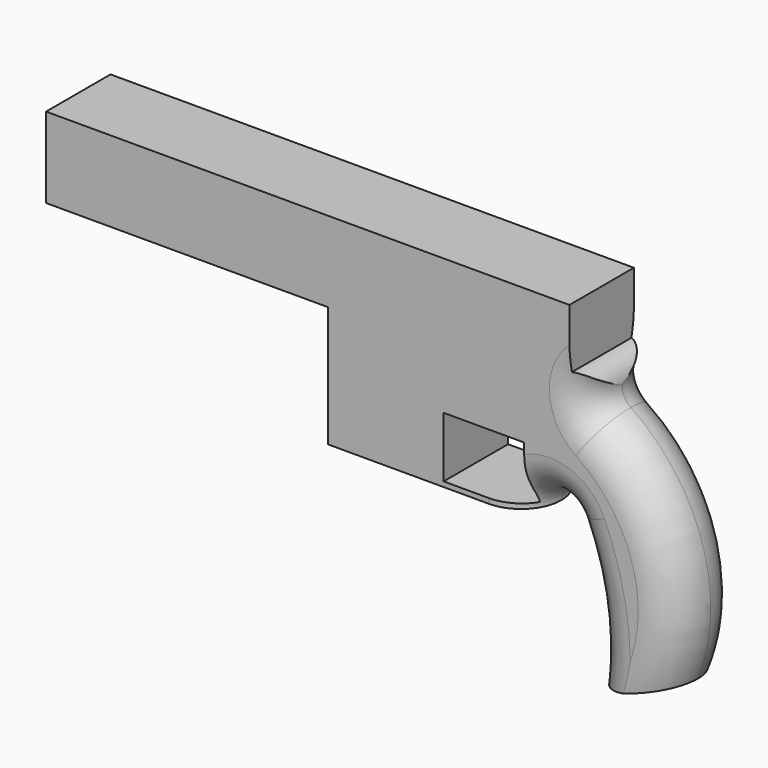
from build123d import *

# Parameters (mm, degrees)
F0_W         = 50.8
F0_H         = 38.1
F1_DEPTH     = 50.8
F2_T2_ANGLE  = 53.6002837339
F2_T4_ANGLE  = 53.6002837339
F2_T6_ANGLE  = 109.3939294159
F2_T8_ANGLE  = 109.3939294159
F2_T10_ANGLE = 342.5650608066
F2_T12_ANGLE = 342.5650608066
F2_T14_ANGLE = 359.64
F2_T16_ANGLE = 359.64


# Not quite as in the source:
# - a fillet or chamfer that OpenCascade refuses, or shapes differently, is made with other operations: its cross-section is extruded or revolved along the edge and cut away or added


with BuildPart() as f1:
    # F0 (on Front) → F1 (new body)
    with BuildSketch(Plane.XZ):
        with BuildLine():
            Line((-177.8, 0), (0, 0))
            Line((0, 0), (0, -76.2))
            Line((0, -76.2), (127, -76.2))
            ThreePointArc((127, -76.2), (137.069140052, -63.7754848813), (151.3100119581, -71.0524158741))
            ThreePointArc((151.3100119581, -71.0524158741), (163.8205179064, -114.6223435958), (164.0100119581, -159.9524158741))
            Line((164.0100119581, -159.9524158741), (213.1969004549, -147.2524158741))
            ThreePointArc((213.1969004549, -147.2524158741), (216.0088779453, -71.4162966266), (170.7058872965, -10.53392448))
            ThreePointArc((170.7058872965, -10.53392448), (166.5887281869, -5.9663543586), (165.1, 0))
            ThreePointArc((165.1, 0), (161.3802561211, 8.9802561211), (152.4, 12.7))
            Line((152.4, 12.7), (152.4, 50.8))
            Line((152.4, 50.8), (-177.8, 50.8))
            Line((-177.8, 50.8), (-177.8, 0))
        make_face()
        with Locations((98.425, -53.975)):
            Rectangle(F0_W, F0_H, mode=Mode.SUBTRACT)
    extrude(amount=F1_DEPTH)

    # F2: fillet of radius 25.4 on 8 edges, made by hand

    # F2_s1 → F2_t2 (revolve, cut)
    with BuildSketch(Plane(origin=(51.1854271814, 0, -115.4451111674), x_dir=(0, 1, 0), z_dir=(-0.4053215847, 0, 0.9141741699))):
        with BuildLine():
            ThreePointArc((-25.4, -109.5246267837), (-43.3605122421, -116.9641145416), (-50.8, -134.9246267837))
            Line((-50.8, -134.9246267837), (-50.8, -109.5246267837))
            Line((-50.8, -109.5246267837), (-25.4, -109.5246267837))
        make_face()
    revolve(axis=Axis((0.3798565029, -50.8, -137.9710095106), (0, 1, 0)), revolution_arc=F2_T2_ANGLE, mode=Mode.SUBTRACT)

    # F2_s3 → F2_t4 (revolve, cut)
    with BuildSketch(Plane(origin=(51.1854271814, 0, -115.4451111674), x_dir=(0, 1, 0), z_dir=(-0.4053215847, 0, 0.9141741699))):
        with BuildLine():
            ThreePointArc((-25.4, -109.5246267837), (-7.4394877579, -116.9641145416), (0, -134.9246267837))
            Line((0, -134.9246267837), (0, -109.5246267837))
            Line((0, -109.5246267837), (-25.4, -109.5246267837))
        make_face()
    revolve(axis=Axis((0.3798565029, 0, -137.9710095106), (0, 1, 0)), revolution_arc=F2_T4_ANGLE, mode=Mode.SUBTRACT)

    # F2_s5 → F2_t6 (revolve, cut)
    with BuildSketch(Plane(origin=(18.3403057366, 0, 13.6443784603), x_dir=(0, 1, 0), z_dir=(-0.802321654, 0, -0.5968919194))):
        with BuildLine():
            ThreePointArc((-25.4, 262.599154914), (-43.3605122421, 255.1596671561), (-50.8, 237.199154914))
            Line((-50.8, 237.199154914), (-50.8, 262.599154914))
            Line((-50.8, 262.599154914), (-25.4, 262.599154914))
        make_face()
    revolve(axis=Axis((106.8588729648, -50.8, -105.3392447997), (0, -1, 0)), revolution_arc=F2_T6_ANGLE, mode=Mode.SUBTRACT)

    # F2_s7 → F2_t8 (revolve, cut)
    with BuildSketch(Plane(origin=(18.3403057366, 0, 13.6443784603), x_dir=(0, 1, 0), z_dir=(-0.802321654, 0, -0.5968919194))):
        with BuildLine():
            ThreePointArc((-25.4, 262.599154914), (-7.4394877579, 255.1596671561), (0, 237.199154914))
            Line((0, 237.199154914), (0, 262.599154914))
            Line((0, 262.599154914), (-25.4, 262.599154914))
        make_face()
    revolve(axis=Axis((106.8588729648, 0, -105.3392447997), (0, -1, 0)), revolution_arc=F2_T8_ANGLE, mode=Mode.SUBTRACT)

    # F2_s9 → F2_t10 (revolve, cut)
    with BuildSketch(Plane(origin=(122.3220401021, 0, -82.378257055), x_dir=(0, 1, 0), z_dir=(0.8294428724, 0, -0.5585915515))):
        with BuildLine():
            ThreePointArc((-25.4, 86.6175778493), (-7.4394877579, 79.1780900914), (0, 61.2175778493))
            Line((0, 61.2175778493), (0, 86.6175778493))
            Line((0, 86.6175778493), (-25.4, 86.6175778493))
        make_face()
    revolve(axis=Axis((177.8, 0, 0), (0, 1, 0)), revolution_arc=F2_T10_ANGLE, mode=Mode.SUBTRACT)

    # F2_s11 → F2_t12 (revolve, cut)
    with BuildSketch(Plane(origin=(122.3220401021, 0, -82.378257055), x_dir=(0, 1, 0), z_dir=(0.8294428724, 0, -0.5585915515))):
        with BuildLine():
            ThreePointArc((-25.4, 86.6175778493), (-43.3605122421, 79.1780900914), (-50.8, 61.2175778493))
            Line((-50.8, 61.2175778493), (-50.8, 86.6175778493))
            Line((-50.8, 86.6175778493), (-25.4, 86.6175778493))
        make_face()
    revolve(axis=Axis((177.8, -50.8, 0), (0, 1, 0)), revolution_arc=F2_T12_ANGLE, mode=Mode.SUBTRACT)

    # F2_s13 → F2_t14 (revolve, cut)
    with BuildSketch(Plane(origin=(50.2149791059, 0, -115.2044645561), x_dir=(0, 1, 0), z_dir=(-0.3995696961, 0, 0.9167028188))):
        with BuildLine():
            ThreePointArc((-25.4, -110.3161729414), (-7.4394877579, -117.7556606993), (0, -135.7161729414))
            Line((0, -135.7161729414), (0, -110.3161729414))
            Line((0, -110.3161729414), (-25.4, -110.3161729414))
        make_face()
    revolve(axis=Axis((139.7, 0, -76.2), (0, 1, 0)), revolution_arc=F2_T14_ANGLE, mode=Mode.SUBTRACT)

    # F2_s15 → F2_t16 (revolve, cut)
    with BuildSketch(Plane(origin=(50.2149791059, 0, -115.2044645561), x_dir=(0, 1, 0), z_dir=(-0.3995696961, 0, 0.9167028188))):
        with BuildLine():
            ThreePointArc((-25.4, -110.3161729414), (-43.3605122421, -117.7556606993), (-50.8, -135.7161729414))
            Line((-50.8, -135.7161729414), (-50.8, -110.3161729414))
            Line((-50.8, -110.3161729414), (-25.4, -110.3161729414))
        make_face()
    revolve(axis=Axis((139.7, -50.8, -76.2), (0, 1, 0)), revolution_arc=F2_T16_ANGLE, mode=Mode.SUBTRACT)


solid = f1.part
